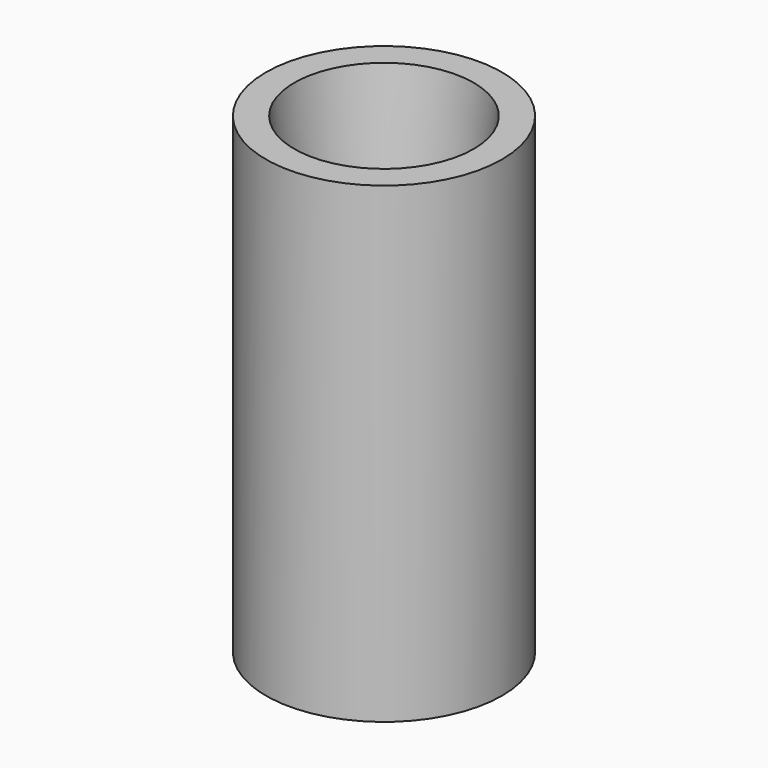
from build123d import *

# Parameters (mm, degrees)
F0_R     = 1.5
F1_DEPTH = 1
F0_R_2   = 2.5
F2_DEPTH = 5
F3_SIZE2 = 0.39999
F3_SIZE  = 3.99999
F4_SIZE2 = 3.99999
F4_SIZE  = 0.39999


# Not quite as in the source:
# - a fillet or chamfer is up to 0.001 mm smaller than in the source, because OpenCascade refuses the exact size


with BuildPart() as f1:
    # F0 (on Top) → F1 (new body, symmetric)
    with BuildSketch(Plane.XY):
        Circle(F0_R)
    extrude(amount=F1_DEPTH, both=True)

    # F0 (on Top) → F2 (join, symmetric)
    with BuildSketch(Plane.XY):
        Circle(F0_R_2)
        Circle(F0_R, mode=Mode.SUBTRACT)
    extrude(amount=F2_DEPTH, both=True)

    # F3 (size 4 and 0.4 in the source; OpenCascade refuses exactly that, so slightly less here)
    f3_edges = [f1.edges().sort_by_distance(p)[0] for p in [
        (-1.5, 0, 5),
    ]]
    f3_side = f1.faces().sort_by_distance((-1.5, 0, 3))[0]
    chamfer(f3_edges, length=F3_SIZE, length2=F3_SIZE2, reference=f3_side)

    # F4 (size 0.4 and 4 in the source; OpenCascade refuses exactly that, so slightly less here)
    f4_edges = [f1.edges().sort_by_distance(p)[0] for p in [
        (-1.5, 0, -5),
    ]]
    f4_side = f1.faces().sort_by_distance((-2.429289, 0, -5))[0]
    chamfer(f4_edges, length=F4_SIZE, length2=F4_SIZE2, reference=f4_side)


solid = f1.part
